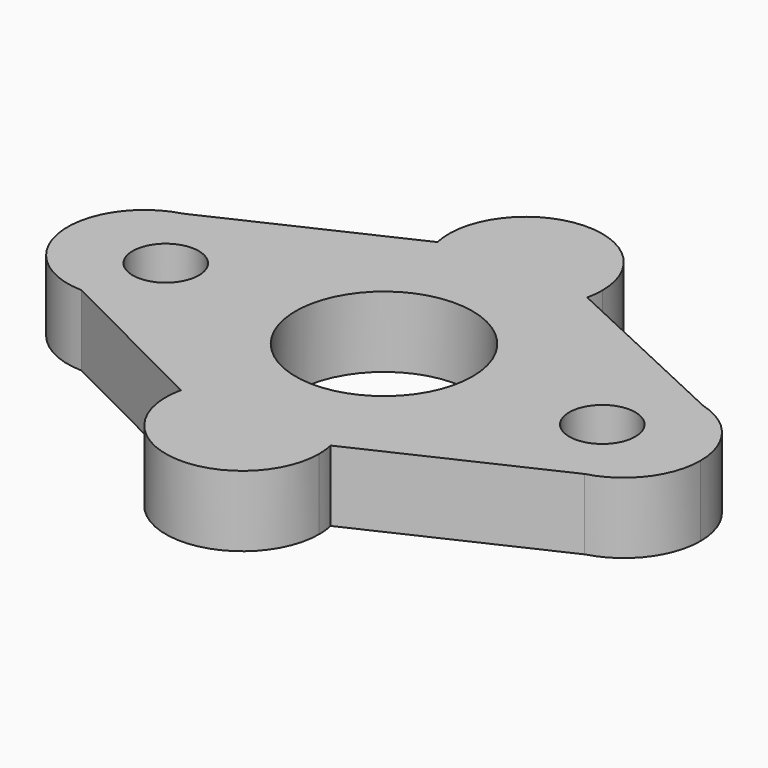
from build123d import *

# Parameters (mm, degrees)
F0_R     = 3.75
F1_DEPTH = 3
F2_R     = 1.4
F3_DEPTH = 6.096


# Not quite as in the source:
# - a feature names something its author has since deleted; it is built from what else it names


with BuildPart() as f1:
    # F0 (on Top) → F1 (new body)
    with BuildSketch(Plane.XY):
        with BuildLine():
            ThreePointArc((-3.1727983399, 6.7958333333), (0, 4.25), (3.1727983399, 6.7958333333))
            ThreePointArc((3.1727983399, 6.7958333333), (0, 7.5), (-3.1727983399, 6.7958333333))
        make_face()
        with BuildLine():
            Line((11.0098453548, 3.1369193284), (3.1727983399, 6.7958333333))
            ThreePointArc((3.1727983399, 6.7958333333), (5.8592267319, 4.6818225195), (7.3284005906, 1.5951629335))
            ThreePointArc((7.3284005906, 1.5951629335), (8.9045755783, 2.9977340645), (11.0098453548, 3.1369193284))
        make_face()
        with BuildLine():
            ThreePointArc((7.3284005906, 1.5951629335), (5.8592267319, 4.6818225195), (3.1727983399, 6.7958333333))
            ThreePointArc((3.1727983399, 6.7958333333), (0, 4.25), (-3.1727983399, 6.7958333333))
            ThreePointArc((-3.1727983399, 6.7958333333), (-5.8592267319, 4.6818225195), (-7.3284005906, 1.5951629335))
            ThreePointArc((-7.3284005906, 1.5951629335), (-7.0163398656, 0.8245610709), (-6.91, 0))
            ThreePointArc((-6.91, 0), (-7.0163398656, -0.8245610709), (-7.3284005906, -1.5951629335))
            ThreePointArc((-7.3284005906, -1.5951629335), (-5.9282154859, -4.5941551076), (-3.3735330862, -6.6984531435))
            ThreePointArc((-3.3735330862, -6.6984531435), (-3.2735278386, -6.7478897064), (-3.1727983399, -6.7958333333))
            ThreePointArc((-3.1727983399, -6.7958333333), (0, -4.25), (3.1727983399, -6.7958333333))
            ThreePointArc((3.1727983399, -6.7958333333), (5.8592267319, -4.6818225195), (7.3284005906, -1.5951629335))
            ThreePointArc((7.3284005906, -1.5951629335), (6.91, 0), (7.3284005906, 1.5951629335))
        make_face()
        Circle(F0_R, mode=Mode.SUBTRACT)
        with BuildLine():
            ThreePointArc((-3.1727983399, 6.7958333333), (0, 7.5), (3.1727983399, 6.7958333333))
            ThreePointArc((3.1727983399, 6.7958333333), (3.2306419335, 7.1458069768), (3.25, 7.5))
            ThreePointArc((3.25, 7.5), (-0.3541930232, 10.7306419335), (-3.1727983399, 6.7958333333))
        make_face()
        with BuildLine():
            ThreePointArc((-7.3284005906, 1.5951629335), (-5.8592267319, 4.6818225195), (-3.1727983399, 6.7958333333))
            Line((-3.1727983399, 6.7958333333), (-11.0098453548, 3.1369193284))
            ThreePointArc((-11.0098453548, 3.1369193284), (-8.9045755783, 2.9977340645), (-7.3284005906, 1.5951629335))
        make_face()
        with BuildLine():
            ThreePointArc((11.0098453548, 3.1369193284), (8.9045755783, 2.9977340645), (7.3284005906, 1.5951629335))
            ThreePointArc((7.3284005906, 1.5951629335), (7.4569767476, 0.8021831371), (7.5, 0))
            ThreePointArc((7.5, 0), (7.4569767476, -0.8021831371), (7.3284005906, -1.5951629335))
            ThreePointArc((7.3284005906, -1.5951629335), (8.9045755783, -2.9977340645), (11.0098453548, -3.1369193284))
            ThreePointArc((11.0098453548, -3.1369193284), (12.7411332204, -1.9749053898), (13.41, 0))
            ThreePointArc((13.41, 0), (12.7411332204, 1.9749053898), (11.0098453548, 3.1369193284))
        make_face()
        with BuildLine():
            ThreePointArc((7.5, 0), (7.4569767476, 0.8021831371), (7.3284005906, 1.5951629335))
            ThreePointArc((7.3284005906, 1.5951629335), (6.91, 0), (7.3284005906, -1.5951629335))
            ThreePointArc((7.3284005906, -1.5951629335), (7.4569767476, -0.8021831371), (7.5, 0))
        make_face()
        with BuildLine():
            ThreePointArc((-6.91, 0), (-7.0163398656, 0.8245610709), (-7.3284005906, 1.5951629335))
            ThreePointArc((-7.3284005906, 1.5951629335), (-7.5, 0), (-7.3284005906, -1.5951629335))
            ThreePointArc((-7.3284005906, -1.5951629335), (-7.0163398656, -0.8245610709), (-6.91, 0))
        make_face()
        with BuildLine():
            ThreePointArc((-7.3284005906, -1.5951629335), (-7.5, 0), (-7.3284005906, 1.5951629335))
            ThreePointArc((-7.3284005906, 1.5951629335), (-8.9045755783, 2.9977340645), (-11.0098453548, 3.1369193284))
            ThreePointArc((-11.0098453548, 3.1369193284), (-13.3855431521, -0.3979590107), (-10.2219168602, -3.2494101468))
            ThreePointArc((-10.2219168602, -3.2494101468), (-8.5469535603, -2.8214501915), (-7.3284005906, -1.5951629335))
        make_face()
        with BuildLine():
            ThreePointArc((11.0098453548, -3.1369193284), (8.9045755783, -2.9977340645), (7.3284005906, -1.5951629335))
            ThreePointArc((7.3284005906, -1.5951629335), (5.8592267319, -4.6818225195), (3.1727983399, -6.7958333333))
            Line((3.1727983399, -6.7958333333), (11.0098453548, -3.1369193284))
        make_face()
        with BuildLine():
            ThreePointArc((-3.3735330862, -6.6984531435), (-5.9282154859, -4.5941551076), (-7.3284005906, -1.5951629335))
            ThreePointArc((-7.3284005906, -1.5951629335), (-8.5469535603, -2.8214501915), (-10.2219168602, -3.2494101468))
            Line((-10.2219168602, -3.2494101468), (-3.3735330862, -6.6984531435))
        make_face()
        with BuildLine():
            ThreePointArc((3.25, -7.5), (3.2306419335, -7.1458069768), (3.1727983399, -6.7958333333))
            ThreePointArc((3.1727983399, -6.7958333333), (0, -7.5), (-3.1727983399, -6.7958333333))
            ThreePointArc((-3.1727983399, -6.7958333333), (-3.1731688138, -6.7975046766), (-3.1735384072, -6.7991762148))
            ThreePointArc((-3.1735384072, -6.7991762148), (-0.3524912598, -10.7308280536), (3.25, -7.5))
        make_face()
        with BuildLine():
            ThreePointArc((-3.1727983399, -6.7958333333), (0, -7.5), (3.1727983399, -6.7958333333))
            ThreePointArc((3.1727983399, -6.7958333333), (0, -4.25), (-3.1727983399, -6.7958333333))
        make_face()
    extrude(amount=F1_DEPTH)

    # F2 (on face) → F3 (cut)
    with BuildSketch(Plane.XY.offset(3)):
        with Locations((-9.25, 0)):
            Circle(F2_R)
        with Locations((9.25, 0)):
            Circle(F2_R)
    extrude(amount=-F3_DEPTH, mode=Mode.SUBTRACT)


solid = f1.part
